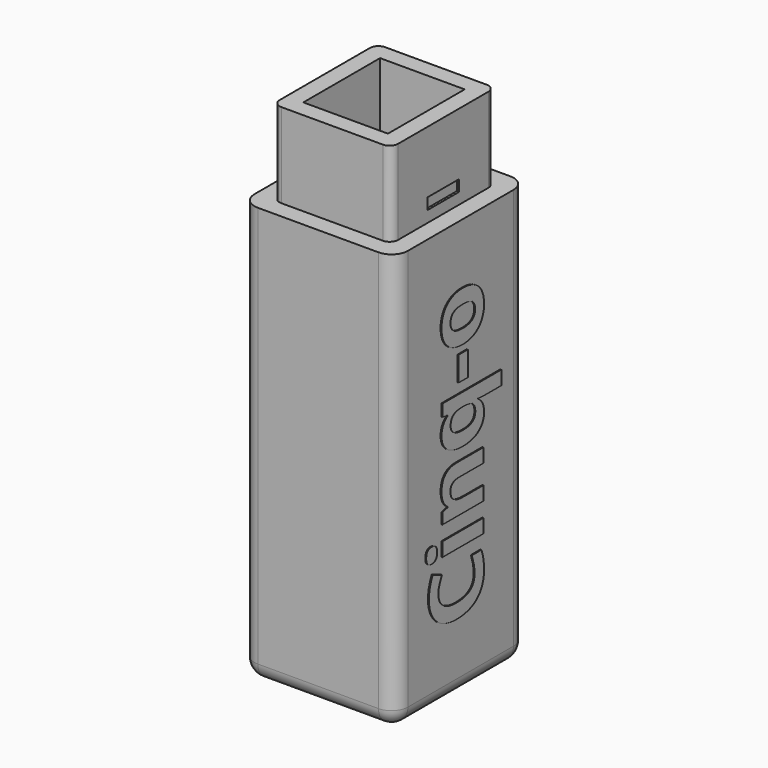
from build123d import *

# Parameters (mm, degrees)
F0_W         = 34.544
F0_H         = 37.084
F1_DEPTH     = 94.107
F2_W         = 26.67
F2_H         = 29.21
F3_DEPTH     = 19.05
F4_W         = 19.05
F4_H         = 21.59
F5_DEPTH     = 109.22
F6_R         = 3.683
F7_R         = 1.905
F8_TEXT_SIZE = 21.1666666667
F9_DEPTH     = 0.2032
F10_W        = 8.89
F10_H        = 2.54
F11_DEPTH    = 0.508
F12_W        = 8.89
F12_H        = 2.54
F13_DEPTH    = 0.508


# Not quite as in the source:
# - Text() gives the source's letters only with a copy of the font that has no kerning and outlines rounded to 1/6400 em; it was checked with that copy


with BuildPart() as f1:
    # F0 (on Top) → F1 (new body)
    with BuildSketch(Plane.XY):
        with Locations((17.272, -18.542)):
            Rectangle(F0_W, F0_H)
    extrude(amount=F1_DEPTH)

    # F2 (on face) → F3 (join)
    with BuildSketch(Plane.XY.offset(94.107)):
        with Locations((17.272, -18.542)):
            Rectangle(F2_W, F2_H)
    extrude(amount=F3_DEPTH)

    # F4 (on face) → F5 (cut)
    with BuildSketch(Plane.XY.offset(113.157)):
        with Locations((17.272, -18.542)):
            Rectangle(F4_W, F4_H)
    extrude(amount=-F5_DEPTH, mode=Mode.SUBTRACT)

    # F6
    f6_edges = [f1.edges().sort_by_distance(p)[0] for p in [
        (34.544, 0, 47.0535),
        (0, 0, 47.0535),
        (34.544, -37.084, 47.0535),
        (34.544, -18.542, 0),
        (17.272, 0, 0),
        (0, -37.084, 47.0535),
        (0, -18.542, 0),
        (17.272, -37.084, 0),
    ]]
    fillet(f6_edges, radius=F6_R)

    # F7
    f7_edges = [f1.edges().sort_by_distance(p)[0] for p in [
        (30.607, -3.937, 103.632),
        (30.607, -33.147, 103.632),
        (3.937, -3.937, 103.632),
        (3.937, -33.147, 103.632),
    ]]
    fillet(f7_edges, radius=F7_R)

    # F8 (on face) → F9 (join)
    with BuildSketch(Plane.YZ.offset(34.544)):
        with Locations(Location((-12.4332935313, 14.4415988146), (0, 0, 90))):
            Text('Cinq-o', F8_TEXT_SIZE, font='Open Sans', font_style=FontStyle.BOLD, text_align=(TextAlign.LEFT, TextAlign.BOTTOM))
    extrude(amount=F9_DEPTH)

    # F10 (on face) → F11 (cut)
    with BuildSketch(Plane.YZ.offset(30.607)):
        with Locations((-18.542, 97.917)):
            Rectangle(F10_W, F10_H)
    extrude(amount=-F11_DEPTH, mode=Mode.SUBTRACT)

    # F12 (on face) → F13 (cut)
    with BuildSketch(Plane(origin=(3.937, 0, 0), x_dir=(0, -1, 0), z_dir=(-1, 0, 0))):
        with Locations((18.542, 97.917)):
            Rectangle(F12_W, F12_H)
    extrude(amount=-F13_DEPTH, mode=Mode.SUBTRACT)


with BuildPart() as f16_1:
    # F16: copy of F1
    add(f1.part.moved(Location((50.8, 0, 0))))


solid = f1.part
